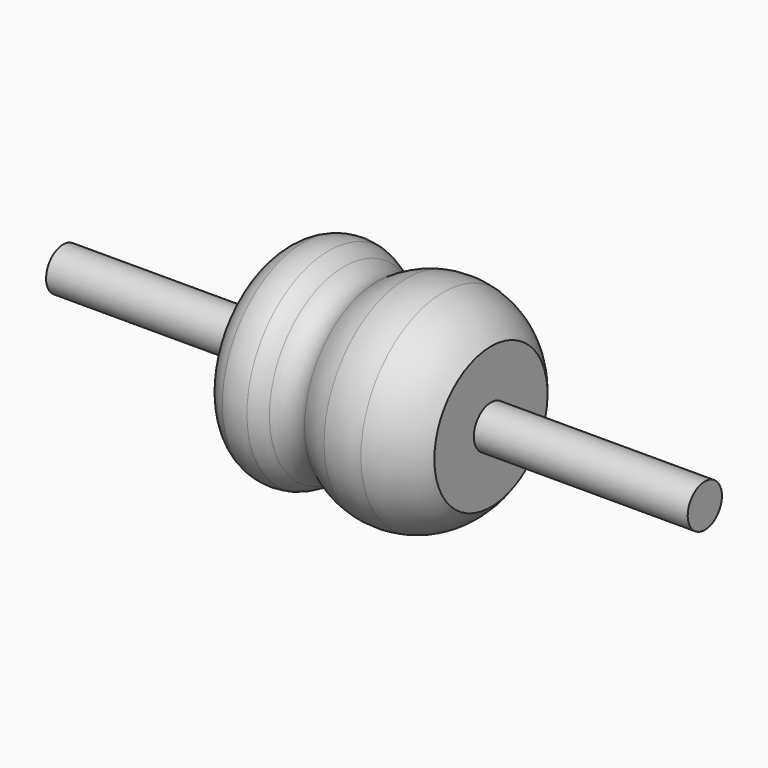
from build123d import *

# Parameters (mm, degrees)
F0_W = 40
F0_H = 4


# Not quite as in the source:
# - a feature names something its author has since deleted; it is built from what else it names
# - the program builds the solid bodies; features that only make, move or delete a surface that nothing else refers to are left out


with BuildPart() as f1:
    # F0 (on Front) → F1 (revolve)
    with BuildSketch(Plane.XZ):
        with Locations((-60, 2)):
            Rectangle(F0_W, F0_H)
        with BuildLine():
            Line((-80, 12.7181895077), (-80, 4))
            Line((-80, 4), (-40, 4))
            Line((-40, 4), (-40, 13.2320560515))
            ThreePointArc((-40, 13.2320560515), (-43.9265726053, 17.0365837136), (-48.9301517038, 19.2403530667))
            ThreePointArc((-48.9301517038, 19.2403530667), (-52.3273584241, 19.6733006707), (-55.7366863479, 19.3493558663))
            ThreePointArc((-55.7366863479, 19.3493558663), (-58.6213477942, 18.4469810503), (-61.2759213851, 17.0017160163))
            ThreePointArc((-61.2759213851, 17.0017160163), (-64.4496036892, 16.152321931), (-67.4653046291, 17.4558853242))
            ThreePointArc((-67.4653046291, 17.4558853242), (-68.8158438678, 18.4427526295), (-70.3514725459, 19.1058573548))
            ThreePointArc((-70.3514725459, 19.1058573548), (-72.7023195146, 19.4301712071), (-75.0368519562, 19.0040031361))
            ThreePointArc((-75.0368519562, 19.0040031361), (-78.4273812016, 16.5787885104), (-80, 12.7181895077))
        make_face()
    revolve(axis=Axis((-60, 0, 0), (1, 0, 0)))


with BuildPart() as f2:
    # F0 (on Front) → F2 (revolve)
    with BuildSketch(Plane.XZ):
        with Locations((-100, 2)):
            Rectangle(F0_W, F0_H)
    revolve(axis=Axis((-60, 0, 0), (1, 0, 0)))


with BuildPart() as f2b:
    # F0 (on Front) → F2, piece 2 (revolve)
    with BuildSketch(Plane.XZ):
        with Locations((-20, 2)):
            Rectangle(F0_W, F0_H)
    revolve(axis=Axis((-60, 0, 0), (1, 0, 0)))


solid = Compound([f1.part, f2.part, f2b.part])
